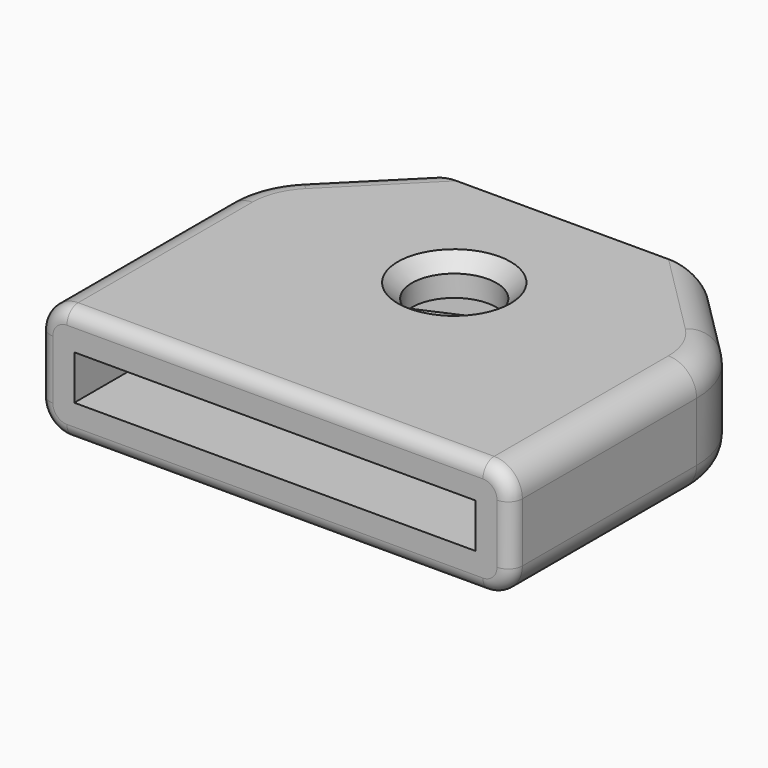
from build123d import *

# Parameters (mm, degrees)
F1_DEPTH = 1.25
F2_T     = 2
F3_R     = 2.38125
F4_DEPTH = 6.501
F6_DEPTH = 3.25
F7_SIZE  = 5.08
F8_R     = 5.08
F9_R     = 1.5875
F10_SIZE = 0.79375
F11_R    = 0.79375


with BuildPart() as f1:
    # F0 (on Top) → F1 (new body, symmetric)
    with BuildSketch(Plane.XY):
        with BuildLine():
            ThreePointArc((1.2815576559, 11.8657501741), (0, 12.1358861541), (-1.2815576559, 11.8657501741))
            Line((-1.2815576559, 11.8657501741), (-8.9015576559, 8.5039854683))
            ThreePointArc((-8.9015576559, 8.5039854683), (-10.2798468525, 7.3328572186), (-10.795, 5.5991214483))
            Line((-10.795, 5.5991214483), (-10.795, -5.5991214483))
            Line((-10.795, -5.5991214483), (10.795, -5.5991214483))
            Line((10.795, -5.5991214483), (10.795, 5.5991214483))
            ThreePointArc((10.795, 5.5991214483), (10.2798468525, 7.3328572186), (8.9015576559, 8.5039854683))
            Line((8.9015576559, 8.5039854683), (1.2815576559, 11.8657501741))
        make_face()
        with BuildLine():
            Line((-8.9015576559, 8.5039854683), (-1.2815576559, 11.8657501741))
            ThreePointArc((-1.2815576559, 11.8657501741), (0, 12.1358861541), (1.2815576559, 11.8657501741))
            Line((1.2815576559, 11.8657501741), (8.9015576559, 8.5039854683))
            ThreePointArc((8.9015576559, 8.5039854683), (10.2798468525, 7.3328572186), (10.795, 5.5991214483))
            Line((10.795, 5.5991214483), (10.795, -5.5991214483))
            Line((10.795, -5.5991214483), (11.295, -5.5991214483))
            Line((11.295, -5.5991214483), (11.295, 5.5991214483))
            ThreePointArc((11.295, 5.5991214483), (10.6987203726, 7.6058864738), (9.1033777592, 8.961444369))
            Line((9.1033777592, 8.961444369), (1.4833777592, 12.3232090749))
            ThreePointArc((1.4833777592, 12.3232090749), (0, 12.6358861541), (-1.4833777592, 12.3232090749))
            Line((-1.4833777592, 12.3232090749), (-9.1033777592, 8.961444369))
            ThreePointArc((-9.1033777592, 8.961444369), (-10.6987203726, 7.6058864738), (-11.295, 5.5991214483))
            Line((-11.295, 5.5991214483), (-11.295, -5.5991214483))
            Line((-11.295, -5.5991214483), (-10.795, -5.5991214483))
            Line((-10.795, -5.5991214483), (-10.795, 5.5991214483))
            ThreePointArc((-10.795, 5.5991214483), (-10.2798468525, 7.3328572186), (-8.9015576559, 8.5039854683))
        make_face()
    extrude(amount=F1_DEPTH, both=True)

    # F2
    f2_openings = [f1.faces().sort_by_distance(p)[0] for p in [
        (0, -5.599121, 0),
    ]]
    offset(amount=F2_T, openings=f2_openings, kind=Kind.INTERSECTION)

    # F3 (on face) → F4 (cut, through all)
    with BuildSketch(Plane(origin=(0, 0, -3.25), x_dir=(1, 0, 0), z_dir=(0, 0, -1))):
        with Locations((0, -7.0158861541)):
            Circle(F3_R)
    extrude(amount=-F4_DEPTH, mode=Mode.SUBTRACT)

    # F5 (on Top) → F6 (join, symmetric)
    with BuildSketch(Plane.XY):
        with BuildLine():
            Line((-9.9106581723, 10.7912799722), (-2.2906581723, 14.1530446781))
            ThreePointArc((-2.2906581723, 14.1530446781), (-1.1704967699, 14.5138639419), (0, 14.6358861541))
            Line((0, 14.6358861541), (-13.295, 14.6358861541))
            Line((-13.295, 14.6358861541), (-13.295, 5.5991214483))
            ThreePointArc((-13.295, 5.5991214483), (-12.3742144529, 8.6980034944), (-9.9106581723, 10.7912799722))
        make_face()
        with BuildLine():
            Line((13.295, 14.6358861541), (0, 14.6358861541))
            ThreePointArc((0, 14.6358861541), (1.1704967699, 14.5138639419), (2.2906581723, 14.1530446781))
            Line((2.2906581723, 14.1530446781), (9.9106581723, 10.7912799722))
            ThreePointArc((9.9106581723, 10.7912799722), (12.3742144529, 8.6980034944), (13.295, 5.5991214483))
            Line((13.295, 5.5991214483), (13.295, 14.6358861541))
        make_face()
    extrude(amount=F6_DEPTH, both=True)

    # F7
    f7_edges = [f1.edges().sort_by_distance(p)[0] for p in [
        (-13.295, 14.635886, 0),
        (13.295, 14.635886, 0),
    ]]
    chamfer(f7_edges, length=F7_SIZE)

    # F8
    f8_edges = [f1.edges().sort_by_distance(p)[0] for p in [
        (-13.295, 9.555886, 0),
        (13.295, 9.555886, 0),
    ]]
    fillet(f8_edges, radius=F8_R)

    # F9
    f9_edges = [f1.edges().sort_by_distance(p)[0] for p in [
        (-13.295, 0.92628, -3.25),
        (-13.295, 0.92628, 3.25),
        (13.295, 0.92628, 3.25),
        (13.295, 0.92628, -3.25),
        (12.908308, 9.395713, -3.25),
        (10.011051, 12.839835, -3.25),
        (-12.908308, 9.395713, -3.25),
        (-10.011051, 12.839835, -3.25),
        (12.908308, 9.395713, 3.25),
        (10.011051, 12.839835, 3.25),
        (-12.908308, 9.395713, 3.25),
        (-10.011051, 12.839835, 3.25),
    ]]
    fillet(f9_edges, radius=F9_R)

    # F10
    f10_edges = [f1.edges().sort_by_distance(p)[0] for p in [
        (-2.38125, 7.015886, -3.25),
        (-2.38125, 7.015886, 3.25),
    ]]
    chamfer(f10_edges, length=F10_SIZE)

    # F11
    f11_edges = [f1.edges().sort_by_distance(p)[0] for p in [
        (0, -5.599121, -3.25),
        (0, -5.599121, 3.25),
        (12.830032, -5.599121, 2.785032),
        (-12.830032, -5.599121, 2.785032),
        (13.295, -5.599121, 0),
        (-13.295, -5.599121, 0),
        (12.830032, -5.599121, -2.785032),
        (-12.830032, -5.599121, -2.785032),
    ]]
    fillet(f11_edges, radius=F11_R)


solid = f1.part
